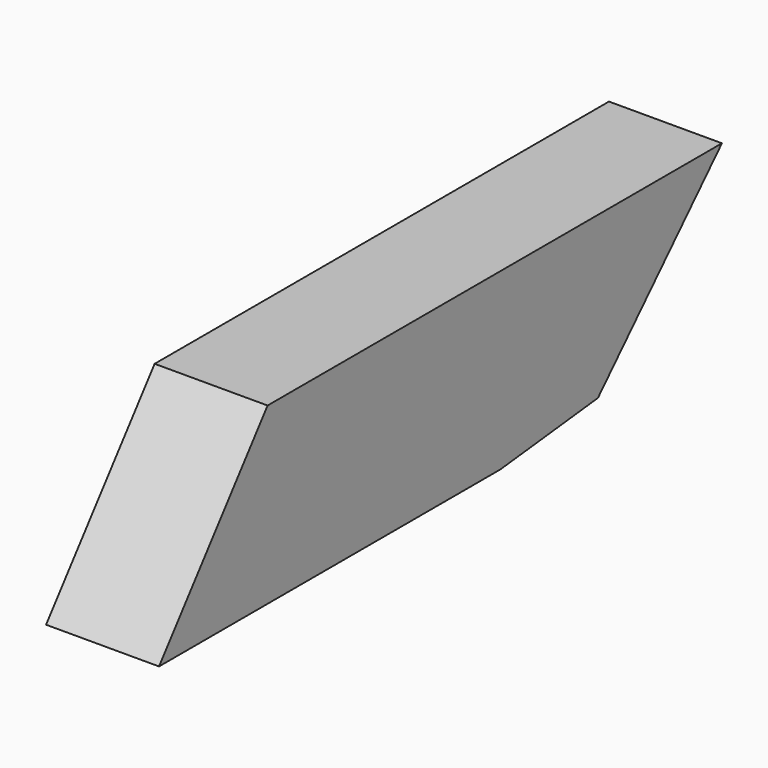
from build123d import *

# Parameters (mm, degrees)
F3_DEPTH = 25.4


# Not quite as in the source:
# - the program builds the solid bodies; features that only make, move or delete a surface that nothing else refers to are left out


with BuildPart() as f3:
    # F2 (on Right) → F3 (new body)
    with BuildSketch(Plane.YZ):
        Polygon((62.2603967786, 39.2553694546), (-65.4462724924, 39.2553694546), (-95.9557369351, 0), (0, 0), (27.4173058569, 3.0065653846), align=None)
    extrude(amount=F3_DEPTH)


solid = f3.part
